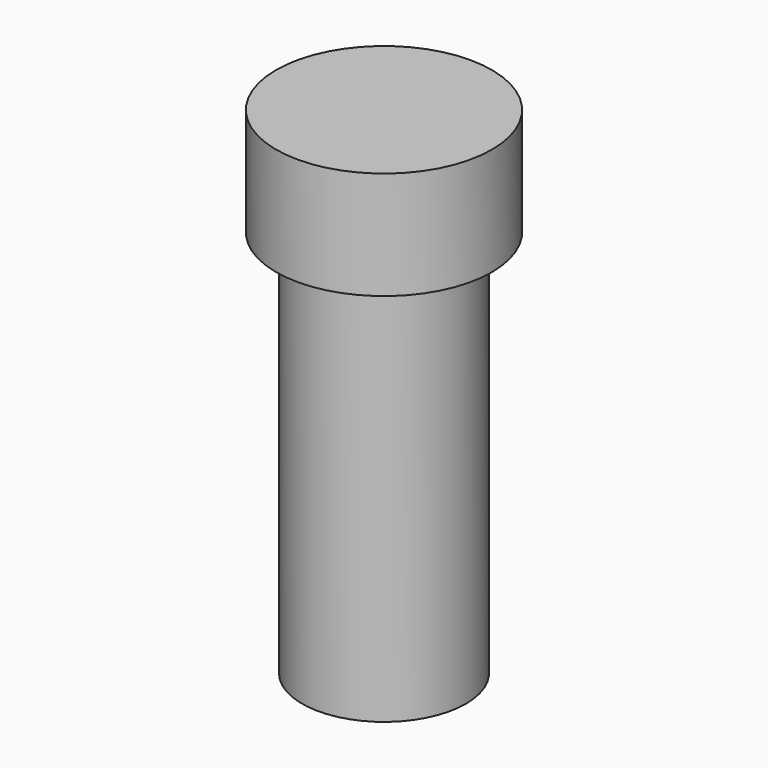
from build123d import *

# Parameters (mm, degrees)
F0_R     = 4.826
F1_DEPTH = 22.86
F2_R     = 6.35
F2_R_2   = 4.826
F3_DEPTH = 6.35
F4_DEPTH = 6.35


# Not quite as in the source:
# - a feature names something its author has since deleted; it is built from what else it names


with BuildPart() as f1:
    # F0 (on Top) → F1 (new body)
    with BuildSketch(Plane.XY):
        Circle(F0_R)
    extrude(amount=F1_DEPTH)

    # F2 (on face) → F3 (join)
    with BuildSketch(Plane.XY.offset(22.86)):
        Circle(F2_R)
        Circle(F2_R_2, mode=Mode.SUBTRACT)
    extrude(amount=F3_DEPTH)

    # F4 (add): a face of the model
    f4_faces = [f1.faces().sort_by_distance(p)[0] for p in [
        (0, 0, 22.86),
    ]]
    extrude(f4_faces, amount=F4_DEPTH)


solid = f1.part
